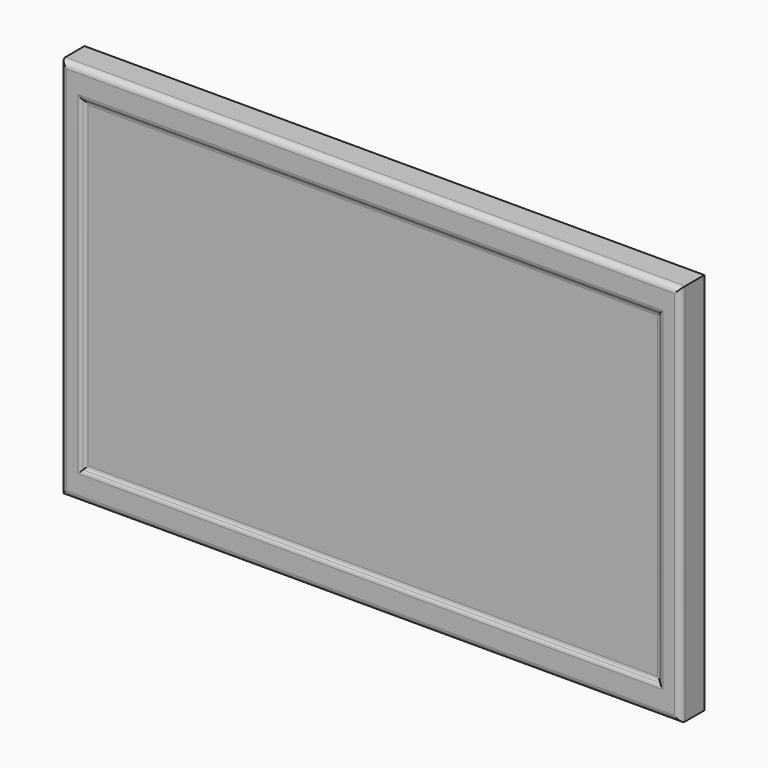
from build123d import *

# Parameters (mm, degrees)
F0_W         = 525.1352317132
F0_H         = 324.7600756863
F0_W_2       = 487.0352317132
F0_H_2       = 273.9600756863
F1_DEPTH     = 25.4
F2_DEPTH     = 22.86
F3_T1_DEPTH  = 550.5352317132
F3_T3_DEPTH  = 350.1600756863
F3_T5_DEPTH  = 487.0352317132
F3_T7_DEPTH  = 273.9600756863
F3_T13_DEPTH = 498.0337543413
F3_T17_DEPTH = 284.9585983143
F3_T24_DEPTH = 498.0337543413
F3_T28_DEPTH = 284.9585983143
F3_T35_DEPTH = 284.9585983143
F3_T39_DEPTH = 498.0337543413
F3_T46_DEPTH = 498.0337543413
F3_T50_DEPTH = 284.9585983143
F4_R         = 5.08
F5_W         = 423.5352317132
F5_H         = 223.1600756863
F6_DEPTH     = 25.4
F6_TAPER     = 45
F7_W         = 133.505359292
F7_H         = 25.4
F8_DEPTH     = 25.4


# Not quite as in the source:
# - a fillet or chamfer that OpenCascade refuses, or shapes differently, is made with other operations: its cross-section is extruded or revolved along the edge and cut away or added


with BuildPart() as f1:
    # F0 (on Front) → F1 (new body)
    with BuildSketch(Plane.XZ):
        Rectangle(F0_W, F0_H)
        Rectangle(F0_W_2, F0_H_2, mode=Mode.SUBTRACT)
    extrude(amount=F1_DEPTH)

    # F0 (on Front) → F2 (join)
    with BuildSketch(Plane.XZ):
        Polygon((-243.5176158566, 136.9800378431), (-243.5176158566, -136.9800378431), (243.5176158566, 136.9800378431), align=None)
        Polygon((-243.5176158566, -136.9800378431), (243.5176158566, -136.9800378431), (243.5176158566, 136.9800378431), align=None)
    extrude(amount=F2_DEPTH)

    # F3: fillet of radius 5.08 on 8 edges, made by hand

    # F3_s2 → F3_t1 (cut)
    with BuildSketch(Plane.YZ.offset(-275.2676158566)):
        with BuildLine():
            ThreePointArc((-20.32, 162.3800378431), (-23.9121024484, 160.8921402916), (-25.4, 157.3000378431))
            Line((-25.4, 157.3000378431), (-25.4, 162.3800378431))
            Line((-25.4, 162.3800378431), (-20.32, 162.3800378431))
        make_face()
        with BuildLine():
            ThreePointArc((-25.4, -157.3000378431), (-23.9121024484, -160.8921402916), (-20.32, -162.3800378431))
            Line((-20.32, -162.3800378431), (-25.4, -162.3800378431))
            Line((-25.4, -162.3800378431), (-25.4, -157.3000378431))
        make_face()
    extrude(amount=F3_T1_DEPTH, mode=Mode.SUBTRACT)

    # F3_s4 → F3_t3 (cut)
    with BuildSketch(Plane.XY.offset(-175.0800378431)):
        with BuildLine():
            ThreePointArc((-262.5676158566, -20.32), (-261.079718305, -23.9121024484), (-257.4876158566, -25.4))
            Line((-257.4876158566, -25.4), (-262.5676158566, -25.4))
            Line((-262.5676158566, -25.4), (-262.5676158566, -20.32))
        make_face()
        with BuildLine():
            ThreePointArc((262.5676158566, -20.32), (261.079718305, -23.9121024484), (257.4876158566, -25.4))
            Line((257.4876158566, -25.4), (262.5676158566, -25.4))
            Line((262.5676158566, -25.4), (262.5676158566, -20.32))
        make_face()
    extrude(amount=F3_T3_DEPTH, mode=Mode.SUBTRACT)

    # F3_s6 → F3_t5 (cut)
    with BuildSketch(Plane.YZ.offset(-243.5176158566)):
        with BuildLine():
            ThreePointArc((-25.4, 141.3794468944), (-24.7194090512, 138.8394468944), (-22.86, 136.9800378431))
            Line((-22.86, 136.9800378431), (-25.4, 136.9800378431))
            Line((-25.4, 136.9800378431), (-25.4, 141.3794468944))
        make_face()
        with BuildLine():
            ThreePointArc((-25.4, -141.3794468944), (-24.7194090512, -138.8394468944), (-22.86, -136.9800378431))
            Line((-22.86, -136.9800378431), (-25.4, -136.9800378431))
            Line((-25.4, -136.9800378431), (-25.4, -141.3794468944))
        make_face()
    extrude(amount=F3_T5_DEPTH, mode=Mode.SUBTRACT)

    # F3_s8 → F3_t7 (cut)
    with BuildSketch(Plane.XY.offset(-136.9800378431)):
        with BuildLine():
            ThreePointArc((247.9170249078, -25.4), (245.3770249078, -24.7194090512), (243.5176158566, -22.86))
            Line((243.5176158566, -22.86), (243.5176158566, -25.4))
            Line((243.5176158566, -25.4), (247.9170249078, -25.4))
        make_face()
        with BuildLine():
            ThreePointArc((-247.9170249078, -25.4), (-245.3770249078, -24.7194090512), (-243.5176158566, -22.86))
            Line((-243.5176158566, -22.86), (-243.5176158566, -25.4))
            Line((-243.5176158566, -25.4), (-247.9170249078, -25.4))
        make_face()
    extrude(amount=F3_T7_DEPTH, mode=Mode.SUBTRACT)


with BuildPart() as f3_tool11:
    # F3_s12 → F3_t13 (new body)
    with BuildSketch(Plane.YZ.offset(-254.5161384847)):
        with BuildLine():
            ThreePointArc((-25.4, 141.3794468944), (-24.7194090512, 138.8394468944), (-22.86, 136.9800378431))
            Line((-22.86, 136.9800378431), (-25.4, 136.9800378431))
            Line((-25.4, 136.9800378431), (-25.4, 141.3794468944))
        make_face()
    extrude(amount=F3_T13_DEPTH)

    split(bisect_by=Plane.YZ.offset(-243.5176158566), keep=Keep.BOTTOM)


with BuildPart() as f3_tool15:
    # F3_s16 → F3_t17 (new body)
    with BuildSketch(Plane.XY.offset(-136.9800378431)):
        with BuildLine():
            ThreePointArc((-247.9170249078, -25.4), (-245.3770249078, -24.7194090512), (-243.5176158566, -22.86))
            Line((-243.5176158566, -22.86), (-243.5176158566, -25.4))
            Line((-243.5176158566, -25.4), (-247.9170249078, -25.4))
        make_face()
    extrude(amount=F3_T17_DEPTH)

    split(bisect_by=Plane.XY.offset(136.9800378431), keep=Keep.TOP)


with BuildPart() as f3_tool11_1:
    add(f3_tool11.part)

    # F3_t19: intersect F3_tool15
    add(f3_tool15.part, mode=Mode.INTERSECT)


with BuildPart() as f1_1:
    add(f1.part)

    # F3_t9: cut F3_tool11
    add(f3_tool11_1.part, mode=Mode.SUBTRACT)


with BuildPart() as f3_tool22:
    # F3_s23 → F3_t24 (new body)
    with BuildSketch(Plane.YZ.offset(-243.5176158566)):
        with BuildLine():
            ThreePointArc((-25.4, 141.3794468944), (-24.7194090512, 138.8394468944), (-22.86, 136.9800378431))
            Line((-22.86, 136.9800378431), (-25.4, 136.9800378431))
            Line((-25.4, 136.9800378431), (-25.4, 141.3794468944))
        make_face()
    extrude(amount=F3_T24_DEPTH)

    split(bisect_by=Plane.YZ.offset(243.5176158566), keep=Keep.TOP)


with BuildPart() as f3_tool26:
    # F3_s27 → F3_t28 (new body)
    with BuildSketch(Plane.XY.offset(147.9785604712)):
        with BuildLine():
            ThreePointArc((247.9170249078, -25.4), (245.3770249078, -24.7194090512), (243.5176158566, -22.86))
            Line((243.5176158566, -22.86), (243.5176158566, -25.4))
            Line((243.5176158566, -25.4), (247.9170249078, -25.4))
        make_face()
    extrude(amount=-F3_T28_DEPTH)

    split(bisect_by=Plane.XY.offset(136.9800378431), keep=Keep.TOP)


with BuildPart() as f3_tool22_1:
    add(f3_tool22.part)

    # F3_t30: intersect F3_tool26
    add(f3_tool26.part, mode=Mode.INTERSECT)


with BuildPart() as f1_2:
    add(f1_1.part)

    # F3_t20: cut F3_tool22
    add(f3_tool22_1.part, mode=Mode.SUBTRACT)


with BuildPart() as f3_tool33:
    # F3_s34 → F3_t35 (new body)
    with BuildSketch(Plane.XY.offset(136.9800378431)):
        with BuildLine():
            ThreePointArc((247.9170249078, -25.4), (245.3770249078, -24.7194090512), (243.5176158566, -22.86))
            Line((243.5176158566, -22.86), (243.5176158566, -25.4))
            Line((243.5176158566, -25.4), (247.9170249078, -25.4))
        make_face()
    extrude(amount=-F3_T35_DEPTH)

    split(bisect_by=Plane.XY.offset(-136.9800378431), keep=Keep.BOTTOM)


with BuildPart() as f3_tool37:
    # F3_s38 → F3_t39 (new body)
    with BuildSketch(Plane.YZ.offset(254.5161384847)):
        with BuildLine():
            ThreePointArc((-25.4, -141.3794468944), (-24.7194090512, -138.8394468944), (-22.86, -136.9800378431))
            Line((-22.86, -136.9800378431), (-25.4, -136.9800378431))
            Line((-25.4, -136.9800378431), (-25.4, -141.3794468944))
        make_face()
    extrude(amount=-F3_T39_DEPTH)

    split(bisect_by=Plane.YZ.offset(243.5176158566), keep=Keep.TOP)


with BuildPart() as f3_tool33_1:
    add(f3_tool33.part)

    # F3_t41: intersect F3_tool37
    add(f3_tool37.part, mode=Mode.INTERSECT)


with BuildPart() as f1_3:
    add(f1_2.part)

    # F3_t31: cut F3_tool33
    add(f3_tool33_1.part, mode=Mode.SUBTRACT)


with BuildPart() as f3_tool44:
    # F3_s45 → F3_t46 (new body)
    with BuildSketch(Plane.YZ.offset(243.5176158566)):
        with BuildLine():
            ThreePointArc((-25.4, -141.3794468944), (-24.7194090512, -138.8394468944), (-22.86, -136.9800378431))
            Line((-22.86, -136.9800378431), (-25.4, -136.9800378431))
            Line((-25.4, -136.9800378431), (-25.4, -141.3794468944))
        make_face()
    extrude(amount=-F3_T46_DEPTH)

    split(bisect_by=Plane.YZ.offset(-243.5176158566), keep=Keep.BOTTOM)


with BuildPart() as f3_tool48:
    # F3_s49 → F3_t50 (new body)
    with BuildSketch(Plane.XY.offset(-147.9785604712)):
        with BuildLine():
            ThreePointArc((-247.9170249078, -25.4), (-245.3770249078, -24.7194090512), (-243.5176158566, -22.86))
            Line((-243.5176158566, -22.86), (-243.5176158566, -25.4))
            Line((-243.5176158566, -25.4), (-247.9170249078, -25.4))
        make_face()
    extrude(amount=F3_T50_DEPTH)

    split(bisect_by=Plane.XY.offset(-136.9800378431), keep=Keep.BOTTOM)


with BuildPart() as f3_tool44_1:
    add(f3_tool44.part)

    # F3_t52: intersect F3_tool48
    add(f3_tool48.part, mode=Mode.INTERSECT)


with BuildPart() as f1_4:
    add(f1_3.part)

    # F3_t42: cut F3_tool44
    add(f3_tool44_1.part, mode=Mode.SUBTRACT)

    # F4
    f4_edges = [f1_4.edges().sort_by_distance(p)[0] for p in [
        (0, -22.86, 136.980038),
        (-243.517616, -22.86, 0),
        (0, -22.86, -136.980038),
        (243.517616, -22.86, 0),
    ]]
    fillet(f4_edges, radius=F4_R)

    # F5 (on face) → F6 (join)
    with BuildSketch(Plane(origin=(0, 0, 0), x_dir=(-1, 0, 0), z_dir=(0, 1, 0))):
        with Locations((0, 25.4)):
            Rectangle(F5_W, F5_H)
    extrude(amount=F6_DEPTH, taper=F6_TAPER)

    # F7 (on face) → F8 (cut)
    with BuildSketch(Plane(origin=(0, 0, 0), x_dir=(-1, 0, 0), z_dir=(0, 1, 0))):
        with Locations((-98.213173449, -73.4800378431)):
            Rectangle(F7_W, F7_H)
    extrude(amount=F8_DEPTH, mode=Mode.SUBTRACT)


solid = f1_4.part
